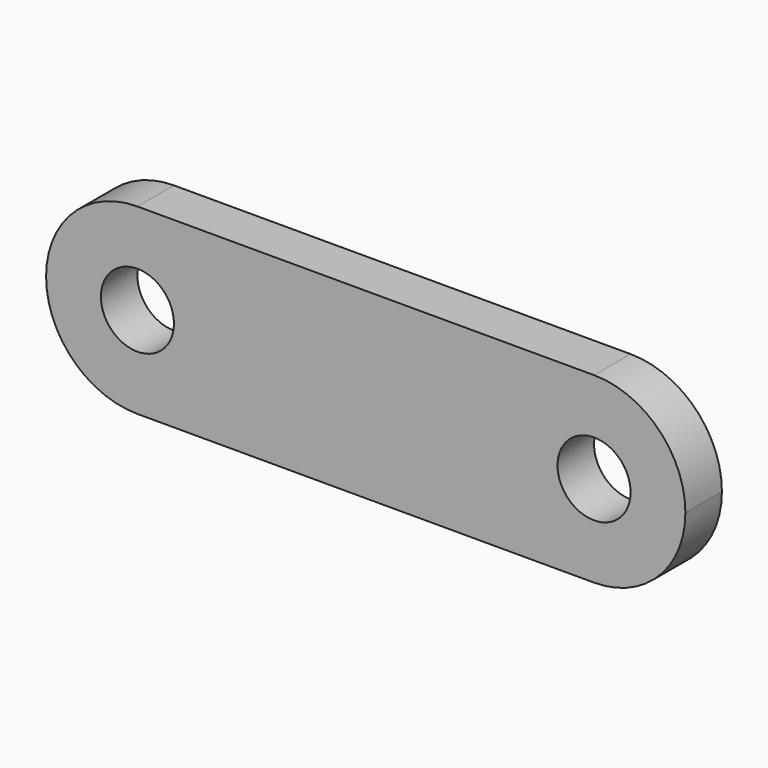
from build123d import *

# Parameters (mm, degrees)
F0_W     = 70
F0_H     = 20
F1_DEPTH = 5
F2_R     = 9.99999
F3_R     = 4
F4_DEPTH = 5.001


# Not quite as in the source:
# - a fillet or chamfer is up to 0.001 mm smaller than in the source, because OpenCascade refuses the exact size


with BuildPart() as f1:
    # F0 (on Front) → F1 (new body)
    with BuildSketch(Plane.XZ):
        with Locations((35, 10)):
            Rectangle(F0_W, F0_H)
    extrude(amount=F1_DEPTH)

    # F2 (radius 10 in the source; OpenCascade refuses exactly that, so slightly less here)
    f2_edges = [f1.edges().sort_by_distance(p)[0] for p in [
        (70, -2.5, 20),
        (70, -2.5, 0),
        (0, -2.5, 20),
        (0, -2.5, 0),
    ]]
    fillet(f2_edges, radius=F2_R)

    # F3 (on face) → F4 (cut, through all)
    with BuildSketch(Plane.XZ.offset(5)):
        with Locations((10, 10)):
            Circle(F3_R)
        with Locations((60, 10)):
            Circle(F3_R)
    extrude(amount=-F4_DEPTH, mode=Mode.SUBTRACT)


solid = f1.part
